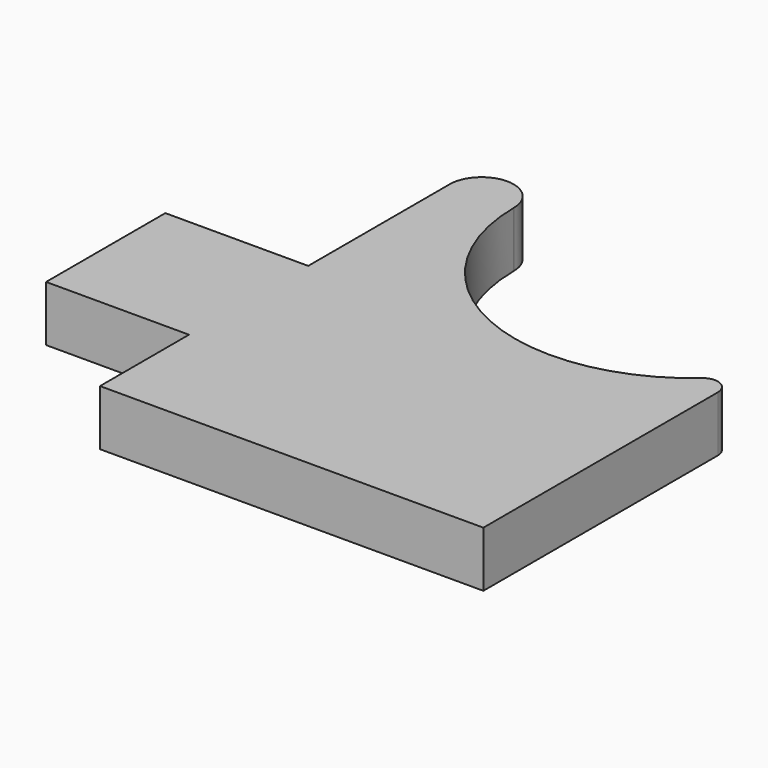
from build123d import *

# Parameters (mm, degrees)
F1_DEPTH = 5
F2_W     = 34.4714387385
F2_H     = 10
F2_W_2   = 12.8498794511
F2_H_2   = 13.4021639824
F3_DEPTH = 5


# Not quite as in the source:
# - ends of sketch curves that miss each other by under 0.0002 mm in the source are joined
# - a feature names something its author has since deleted; it is built from what else it names


with BuildPart() as f1:
    # F0 (on Top) → F1 (new body)
    with BuildSketch(Plane.XY):
        with BuildLine():
            Line((0, 29.2999204248), (0, 0))
            Line((0, 0), (34.4714387385, 0))
            Line((34.4714387385, 0), (34.4714387385, 16.3473710418))
            ThreePointArc((34.4714387385, 16.3473710418), (32.5790927131, 15.1300794804), (32.2559916738, 17.3568210333))
            ThreePointArc((32.2559916738, 17.3568210333), (15.182844974, 14.8438668457), (5.7578901922, 29.2999210911))
            ThreePointArc((5.7578901922, 29.2999210911), (2.8789043427, 26.4210160822), (0, 29.2999204248))
        make_face()
        with BuildLine():
            ThreePointArc((5.7577396052, 29.3198639813), (2.8689325046, 32.1788074974), (0, 29.2999204248))
            ThreePointArc((0, 29.2999204248), (2.8789043427, 26.4210160822), (5.7578086853, 29.2999204248))
            ThreePointArc((5.7578086853, 29.2999204248), (5.7578117914, 29.3098925127), (5.7577396052, 29.3198639813))
        make_face()
        with BuildLine():
            ThreePointArc((32.2559916738, 17.3568210333), (32.5790927131, 15.1300794804), (34.4714387385, 16.3473710418))
            ThreePointArc((34.4714387385, 16.3473710418), (33.6883902233, 17.5646626032), (32.2559916738, 17.3568210333))
        make_face()
    extrude(amount=F1_DEPTH)

    # F2 (on face) → F3 (join)
    with BuildSketch(Plane.XY.offset(5)):
        with BuildLine():
            Line((0, 0), (34.4714387385, 0))
            Line((34.4714387385, 0), (34.4714387385, 16.3473710418))
            ThreePointArc((34.4714387385, 16.3473710418), (33.6883902233, 17.5646626032), (32.2559916738, 17.3568210333))
            ThreePointArc((32.2559916738, 17.3568210333), (15.182844974, 14.8438668457), (5.7578901922, 29.2999210911))
            ThreePointArc((5.7578901922, 29.2999210911), (5.757811792, 29.3098923335), (5.7577396052, 29.3198639813))
            ThreePointArc((5.7577396052, 29.3198639813), (2.8689325046, 32.1788074974), (0, 29.2999204248))
            Line((0, 29.2999204248), (0, 25.4882741719))
            Line((0, 25.4882741719), (0, 13.4021639824))
            Line((0, 13.4021639824), (0, 0))
        make_face()
        with Locations((17.2357193692, -5)):
            Rectangle(F2_W, F2_H)
        with Locations((-6.4249397255, 6.7010819912)):
            Rectangle(F2_W_2, F2_H_2)
    extrude(amount=-F3_DEPTH)


solid = f1.part
